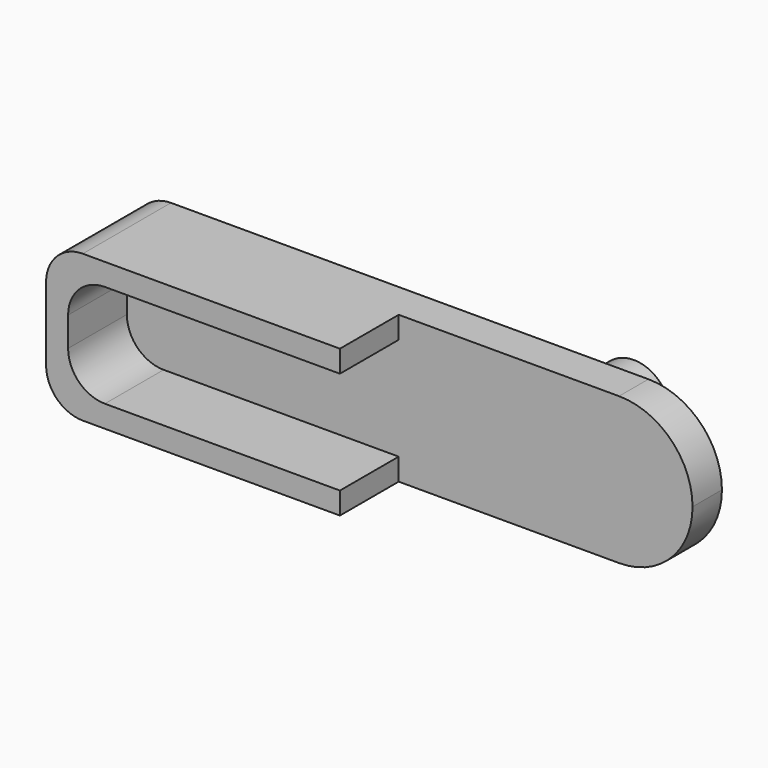
from build123d import *

# Parameters (mm, degrees)
F0_W     = 50.8
F0_H     = 12.7
F1_DEPTH = 3.175
F2_R     = 3.175
F3_DEPTH = 6.35
F5_DEPTH = 6.35
F6_R     = 6.34999
F7_R     = 3.175


# Not quite as in the source:
# - a fillet or chamfer is up to 0.001 mm smaller than in the source, because OpenCascade refuses the exact size


with BuildPart() as f1:
    # F0 (on Front) → F1 (new body)
    with BuildSketch(Plane.XZ):
        with Locations((25.4, 6.35)):
            Rectangle(F0_W, F0_H)
    extrude(amount=F1_DEPTH)

    # F2 (on face) → F3 (join)
    with BuildSketch(Plane(origin=(0, 0, 0), x_dir=(-1, 0, 0), z_dir=(0, 1, 0))):
        with Locations((-38.1, 6.35)):
            Circle(F2_R)
    extrude(amount=F3_DEPTH)

    # F4 (on face) → F5 (join)
    with BuildSketch(Plane.XZ.offset(3.175)):
        Polygon((25.4, 10.795), (25.4, 12.7), (0, 12.7), (0, 0), (25.4, 0), (25.4, 1.905), (1.905, 1.905), (1.905, 10.795), align=None)
    extrude(amount=F5_DEPTH)

    # F6 (radius 6.35 in the source; OpenCascade refuses exactly that, so slightly less here)
    f6_edges = [f1.edges().sort_by_distance(p)[0] for p in [
        (50.8, -1.5875, 0),
        (50.8, -1.5875, 12.7),
    ]]
    fillet(f6_edges, radius=F6_R)

    # F7
    f7_edges = [f1.edges().sort_by_distance(p)[0] for p in [
        (0, -4.7625, 12.7),
        (0, -4.7625, 0),
        (1.905, -6.35, 10.795),
        (1.905, -6.35, 1.905),
    ]]
    fillet(f7_edges, radius=F7_R)


solid = f1.part
